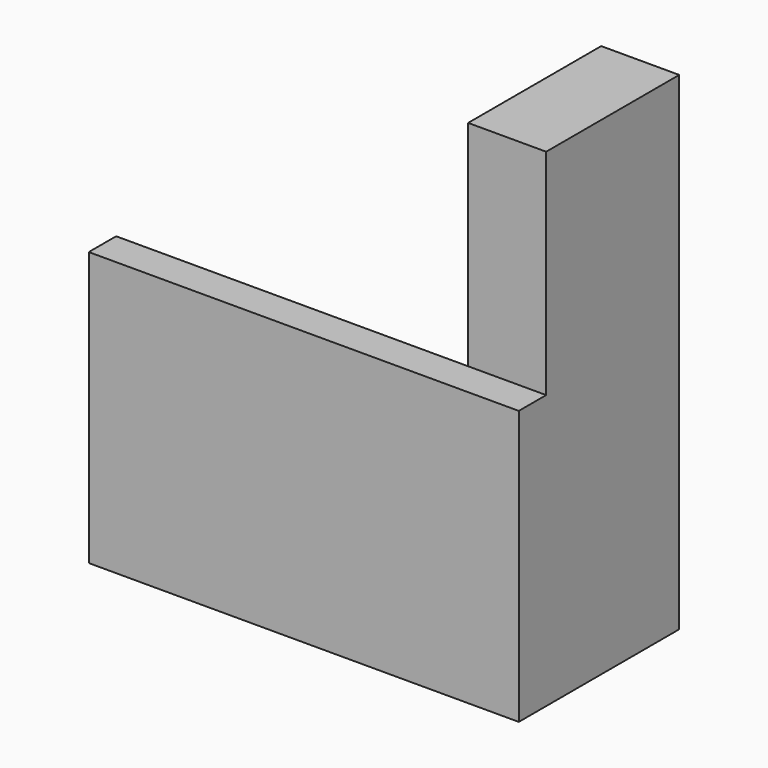
from build123d import *

# Parameters (mm, degrees)
F4_W     = 570
F4_H     = 1215
F5_DEPTH = 1565
F1_E1_W  = 3141
F1_E1_H  = 250
F6_DEPTH = 2000
F7_DEPTH = 2000


# Not quite as in the source:
# - an extrude ends at something that could not be found from the text; its depth is read off the source's solid
# - the program builds the solid bodies; features that only make, move or delete a surface that nothing else refers to are left out


with BuildPart() as f5:
    # F4 (on face) → F5 (new body)
    with BuildSketch(Plane(origin=(0, 0, 0), x_dir=(1, 0, 0), z_dir=(0, 0, -1))):
        with Locations((-285, -607.5)):
            Rectangle(F4_W, F4_H)
    extrude(amount=-F5_DEPTH)

    # F1_E1 (on explicit) → F6 (join)
    with BuildSketch(Plane(origin=(-3141, 0, 0), x_dir=(1, 0, 0), z_dir=(0, 0, -1))):
        with Locations((1570.5, 125)):
            Rectangle(F1_E1_W, F1_E1_H)
    extrude(amount=F6_DEPTH)

    # F7 (add, through all): a face of the model
    f7_faces = [f5.faces().sort_by_distance(p)[0] for p in [
        (-285, 607.5, 0),
    ]]
    extrude(f7_faces, amount=F7_DEPTH)


solid = f5.part
